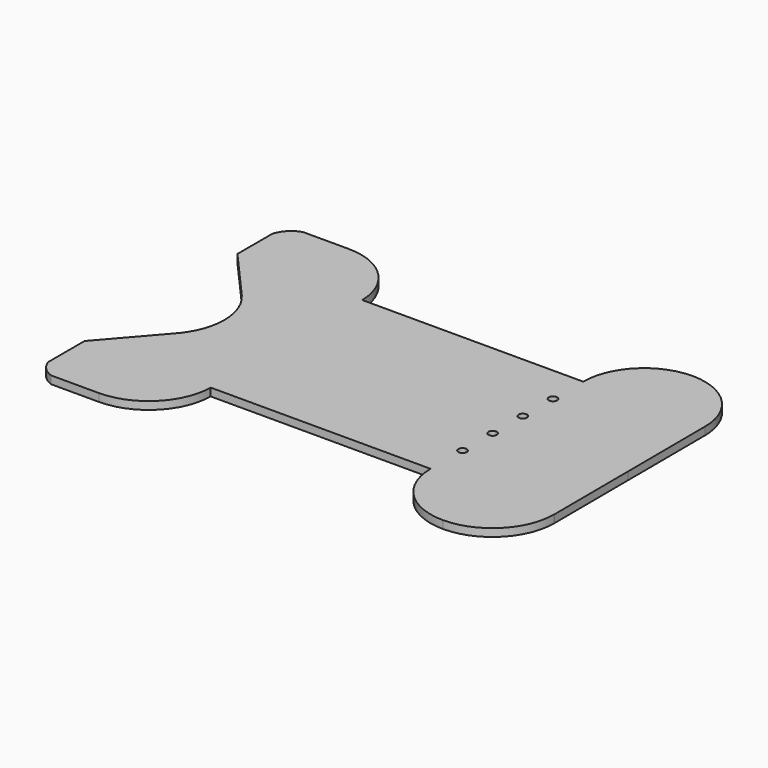
from build123d import *

# Parameters (mm, degrees)
F1_DEPTH = 3.175


# Not quite as in the source:
# - a length typed as a fraction of an inch, garbled in the dataset ("3 / 203.2 mm" for 3/8 in), is restored
# - a feature names something its author has since deleted; it is built from what else it names


with BuildPart() as f1:
    # F0 (on Top) → F1 (new body)
    with BuildSketch(Plane.XY):
        with BuildLine():
            Line((-58.4220365395, 55.6676574051), (-83.8141146934, 55.6676574051))
            Line((-83.8141146934, 55.6676574051), (-83.8141146934, 17.4082663185))
            Line((-83.8141146934, 17.4082663185), (-54.5982423949, 17.2266236973))
            ThreePointArc((-54.5982423949, 17.2266236973), (-52.878445863, 18.9304561303), (-51.1692755304, 17.2159644142))
            ThreePointArc((-51.1692755304, 17.2159644142), (-51.1692838142, 17.2106347468), (-51.1693086658, 17.205305131))
            Line((-51.1693086658, 17.205305131), (-48.1096365395, 17.1862823595))
            Line((-48.1096365395, 17.1862823595), (-48.1096365395, 55.6676574051))
            Line((-48.1096365395, 55.6676574051), (-51.9196365395, 55.6676574051))
            Line((-51.9196365395, 55.6676574051), (-58.4220365395, 55.6676574051))
        make_face()
        with BuildLine():
            Line((-83.8141146934, 80.4333333333), (-83.8141146934, 55.6676574051))
            Line((-83.8141146934, 55.6676574051), (-58.4220365395, 55.6676574051))
            ThreePointArc((-58.4220365395, 55.6676574051), (-66.0792878183, 73.2167300378), (-83.8141146934, 80.4333333333))
        make_face()
        with BuildLine():
            Line((-96.5141146934, 55.6676574051), (-83.8141146934, 55.6676574051))
            Line((-83.8141146934, 55.6676574051), (-83.8141146934, 80.4333333333))
            Line((-83.8141146934, 80.4333333333), (-96.5141146934, 80.4333333333))
            Line((-96.5141146934, 80.4333333333), (-102.2933936502, 80.4333333333))
            ThreePointArc((-102.2933936502, 80.4333333333), (-106.1483818555, 78.2913178986), (-108.7325867358, 74.7176574051))
            Line((-108.7325867358, 74.7176574051), (-102.8641146934, 74.7176574051))
            Line((-102.8641146934, 74.7176574051), (-99.6891146934, 74.7176574051))
            Line((-99.6891146934, 74.7176574051), (-99.6891146934, 55.6676574051))
            Line((-99.6891146934, 55.6676574051), (-96.5141146934, 55.6676574051))
        make_face()
        with BuildLine():
            Line((-83.8141146934, 17.4082663185), (-83.8141146934, 55.6676574051))
            Line((-83.8141146934, 55.6676574051), (-96.5141146934, 55.6676574051))
            Line((-96.5141146934, 55.6676574051), (-99.6891146934, 55.6676574051))
            Line((-99.6891146934, 55.6676574051), (-102.8641146934, 55.6676574051))
            Line((-102.8641146934, 55.6676574051), (-109.2141146934, 55.6676574051))
            Line((-109.2141146934, 55.6676574051), (-90.4137483739, 34.3826312783))
            ThreePointArc((-90.4137483739, 34.3826312783), (-85.6948772916, 26.5569289565), (-84.0509922302, 17.5676574051))
            ThreePointArc((-84.0509922302, 17.5676574051), (-84.0511149543, 17.4886993707), (-84.0514831256, 17.4097420993))
            Line((-84.0514831256, 17.4097420993), (-83.8141146934, 17.4082663185))
        make_face()
        with BuildLine():
            Line((-54.5982423949, 17.2266236973), (-83.8141146934, 17.4082663185))
            Line((-83.8141146934, 17.4082663185), (-83.8141146934, -21.4370436153))
            Line((-83.8141146934, -21.4370436153), (-58.4141146934, -21.4370436153))
            Line((-58.4141146934, -21.4370436153), (-48.1096365395, -21.4370436153))
            Line((-48.1096365395, -21.4370436153), (-48.1096365395, 17.1862823595))
            Line((-48.1096365395, 17.1862823595), (-51.1693086658, 17.205305131))
            ThreePointArc((-51.1693086658, 17.205305131), (-52.8944348135, 15.5014975496), (-54.5982423949, 17.2266236973))
        make_face()
        with BuildLine():
            Line((-83.8141146934, -21.4370436153), (-83.8141146934, 17.4082663185))
            Line((-83.8141146934, 17.4082663185), (-84.0514831256, 17.4097420993))
            ThreePointArc((-84.0514831256, 17.4097420993), (-85.9174728188, 8.0108031049), (-91.1328551507, -0.0279629004))
            Line((-91.1328551507, -0.0279629004), (-91.0666517454, 0))
            Line((-91.0666517454, 0), (-109.6934945268, -21.4370436153))
            Line((-109.6934945268, -21.4370436153), (-103.5974945268, -21.4370436153))
            Line((-103.5974945268, -21.4370436153), (-100.1684945268, -21.4370436153))
            Line((-100.1684945268, -21.4370436153), (-83.8141146934, -21.4370436153))
        make_face()
        with BuildLine():
            Line((-58.4141146934, -21.4370436153), (-83.8141146934, -21.4370436153))
            Line((-83.8141146934, -21.4370436153), (-83.8141146934, -46.5666666667))
            ThreePointArc((-83.8141146934, -46.5666666667), (-65.9485232906, -39.2230246493), (-58.4141146934, -21.4370436153))
        make_face()
        with BuildLine():
            Line((-83.8141146934, -46.5666666667), (-83.8141146934, -21.4370436153))
            Line((-83.8141146934, -21.4370436153), (-100.1684945268, -21.4370436153))
            Line((-100.1684945268, -21.4370436153), (-100.1684945268, -40.4870436153))
            Line((-100.1684945268, -40.4870436153), (-103.5974945268, -40.4870436153))
            Line((-103.5974945268, -40.4870436153), (-109.4795895949, -40.4870436153))
            ThreePointArc((-109.4795895949, -40.4870436153), (-107.0154315461, -44.2413370786), (-103.1736042979, -46.5666666667))
            Line((-103.1736042979, -46.5666666667), (-96.7538046101, -46.5666666667))
            Line((-96.7538046101, -46.5666666667), (-83.8141146934, -46.5666666667))
        make_face()
        with BuildLine():
            ThreePointArc((-51.1692755304, 17.2159644142), (-52.878445863, 18.9304561303), (-54.5982423949, 17.2266236973))
            Line((-54.5982423949, 17.2266236973), (-51.1693086658, 17.205305131))
            ThreePointArc((-51.1693086658, 17.205305131), (-51.1692838142, 17.2106347468), (-51.1692755304, 17.2159644142))
        make_face()
        with BuildLine():
            Line((-51.1693086658, 17.205305131), (-54.5982423949, 17.2266236973))
            ThreePointArc((-54.5982423949, 17.2266236973), (-52.8944348135, 15.5014975496), (-51.1693086658, 17.205305131))
        make_face()
        with BuildLine():
            Line((56.1858853066, 55.6676574051), (56.1858853066, 80.4333333333))
            ThreePointArc((56.1858853066, 80.4333333333), (38.6739079171, 73.1796347946), (31.4202093784, 55.6676574051))
            Line((31.4202093784, 55.6676574051), (56.1858853066, 55.6676574051))
        make_face()
        with BuildLine():
            ThreePointArc((80.9515612348, 55.6676574051), (73.6978626961, 73.1796347946), (56.1858853066, 80.4333333333))
            Line((56.1858853066, 80.4333333333), (56.1858853066, 55.6676574051))
            Line((56.1858853066, 55.6676574051), (80.9515612348, 55.6676574051))
        make_face()
        with BuildLine():
            Line((-102.8641146934, 55.6676574051), (-99.6891146934, 55.6676574051))
            Line((-99.6891146934, 55.6676574051), (-99.6891146934, 74.7176574051))
            Line((-99.6891146934, 74.7176574051), (-102.8641146934, 74.7176574051))
            Line((-102.8641146934, 74.7176574051), (-102.8641146934, 71.6696574051))
            ThreePointArc((-102.8641146934, 71.6696574051), (-101.651780117, 71.1674919815), (-101.1496146934, 69.9551574051))
            ThreePointArc((-101.1496146934, 69.9551574051), (-101.651780117, 68.7428228288), (-102.8641146934, 68.2406574051))
            Line((-102.8641146934, 68.2406574051), (-102.8641146934, 62.1446574051))
            ThreePointArc((-102.8641146934, 62.1446574051), (-101.651780117, 61.6424919815), (-101.1496146934, 60.4301574051))
            ThreePointArc((-101.1496146934, 60.4301574051), (-101.651780117, 59.2178228288), (-102.8641146934, 58.7156574051))
            Line((-102.8641146934, 58.7156574051), (-102.8641146934, 55.6676574051))
        make_face()
        with BuildLine():
            Line((-100.1684945268, -40.4870436153), (-100.1684945268, -21.4370436153))
            Line((-100.1684945268, -21.4370436153), (-103.5974945268, -21.4370436153))
            Line((-103.5974945268, -21.4370436153), (-103.5974945268, -25.4485957723))
            ThreePointArc((-103.5974945268, -25.4485957723), (-102.3851599505, -25.9507611959), (-101.8829945268, -27.1630957723))
            ThreePointArc((-101.8829945268, -27.1630957723), (-102.3851599505, -28.3754303486), (-103.5974945268, -28.8775957723))
            Line((-103.5974945268, -28.8775957723), (-103.5974945268, -32.9818256598))
            ThreePointArc((-103.5974945268, -32.9818256598), (-102.3851599505, -33.4839910834), (-101.8829945268, -34.6963256598))
            ThreePointArc((-101.8829945268, -34.6963256598), (-102.3851599505, -35.9086602361), (-103.5974945268, -36.4108256598))
            Line((-103.5974945268, -36.4108256598), (-103.5974945268, -40.4870436153))
            Line((-103.5974945268, -40.4870436153), (-100.1684945268, -40.4870436153))
        make_face()
        Polygon((-39.2196365395, 55.6676574051), (-48.1096365395, 55.6676574051), (-48.1096365395, 17.1862823595), (-39.2196365395, 17.1310109342), align=None)
        with BuildLine():
            Line((81.1369927167, 16.382722696), (80.9515612348, 55.6676574051))
            ThreePointArc((80.9515612348, 55.6676574051), (73.6978626961, 38.1556800156), (56.1858853066, 30.9019814769))
            Line((56.1858853066, 30.9019814769), (56.1858853066, 26.6474814769))
            ThreePointArc((56.1858853066, 26.6474814769), (57.398219883, 26.1453160533), (57.9003853066, 24.9329814769))
            ThreePointArc((57.9003853066, 24.9329814769), (57.398219883, 23.7206469006), (56.1858853066, 23.2184814769))
            Line((56.1858853066, 23.2184814769), (56.1858853066, 16.5378501727))
            Line((56.1858853066, 16.5378501727), (81.1369927167, 16.382722696))
        make_face()
        with BuildLine():
            ThreePointArc((56.1858853066, 30.9019814769), (73.6978626961, 38.1556800156), (80.9515612348, 55.6676574051))
            Line((80.9515612348, 55.6676574051), (56.1858853066, 55.6676574051))
            Line((56.1858853066, 55.6676574051), (56.1858853066, 30.9019814769))
        make_face()
        with BuildLine():
            Line((31.35631828, 42.1423083088), (31.4202093784, 55.6676574051))
            Line((31.4202093784, 55.6676574051), (24.2803634605, 55.6676574051))
            Line((24.2803634605, 55.6676574051), (20.4703634605, 55.6676574051))
            Line((20.4703634605, 55.6676574051), (20.4703634605, 16.7599027932))
            Line((20.4703634605, 16.7599027932), (23.5155513145, 16.7409700741))
            ThreePointArc((23.5155513145, 16.7409700741), (25.2353478464, 18.4448025071), (26.944518179, 16.730310791))
            ThreePointArc((26.944518179, 16.730310791), (26.9445098952, 16.7249811236), (26.9444850436, 16.7196515078))
            Line((26.9444850436, 16.7196515078), (31.2361005906, 16.6929694259))
            Line((31.2361005906, 16.6929694259), (31.2681297634, 23.4733465661))
            ThreePointArc((31.2681297634, 23.4733465661), (29.5617477636, 25.1959263091), (31.2843275066, 26.9023083088))
            Line((31.2843275066, 26.9023083088), (31.3401205367, 38.7133465661))
            ThreePointArc((31.3401205367, 38.7133465661), (29.633738537, 40.4359263091), (31.35631828, 42.1423083088))
        make_face()
        with BuildLine():
            Line((56.1858853066, 55.6676574051), (31.4202093784, 55.6676574051))
            ThreePointArc((31.4202093784, 55.6676574051), (38.6739079171, 38.1556800156), (56.1858853066, 30.9019814769))
            Line((56.1858853066, 30.9019814769), (56.1858853066, 55.6676574051))
        make_face()
        with BuildLine():
            ThreePointArc((56.1858853066, 30.9019814769), (38.6739079171, 38.1556800156), (31.4202093784, 55.6676574051))
            Line((31.4202093784, 55.6676574051), (31.35631828, 42.1423083088))
            ThreePointArc((31.35631828, 42.1423083088), (32.5634139947, 41.6372952408), (33.0627194083, 40.4278274374))
            ThreePointArc((33.0627194083, 40.4278274374), (32.5576872116, 39.2126328511), (31.3401205367, 38.7133465661))
            Line((31.3401205367, 38.7133465661), (31.2843275066, 26.9023083088))
            ThreePointArc((31.2843275066, 26.9023083088), (32.4914232214, 26.3972952408), (32.990728635, 25.1878274374))
            ThreePointArc((32.990728635, 25.1878274374), (32.4856964383, 23.9726328511), (31.2681297634, 23.4733465661))
            Line((31.2681297634, 23.4733465661), (31.2361005906, 16.6929694259))
            Line((31.2361005906, 16.6929694259), (56.1858853066, 16.5378501727))
            Line((56.1858853066, 16.5378501727), (56.1858853066, 23.2184814769))
            ThreePointArc((56.1858853066, 23.2184814769), (54.4713853066, 24.9329814769), (56.1858853066, 26.6474814769))
            Line((56.1858853066, 26.6474814769), (56.1858853066, 30.9019814769))
        make_face()
        with BuildLine():
            Line((-109.2141146934, 55.6676574051), (-102.8641146934, 55.6676574051))
            Line((-102.8641146934, 55.6676574051), (-102.8641146934, 58.7156574051))
            ThreePointArc((-102.8641146934, 58.7156574051), (-104.5786146934, 60.4301574051), (-102.8641146934, 62.1446574051))
            Line((-102.8641146934, 62.1446574051), (-102.8641146934, 68.2406574051))
            ThreePointArc((-102.8641146934, 68.2406574051), (-104.5786146934, 69.9551574051), (-102.8641146934, 71.6696574051))
            Line((-102.8641146934, 71.6696574051), (-102.8641146934, 74.7176574051))
            Line((-102.8641146934, 74.7176574051), (-108.7325867358, 74.7176574051))
            ThreePointArc((-108.7325867358, 74.7176574051), (-108.9982771043, 74.0351876591), (-109.2141146934, 73.3353516345))
            Line((-109.2141146934, 73.3353516345), (-109.2141146934, 68.0504953692))
            Line((-109.2141146934, 68.0504953692), (-109.2141146934, 55.6676574051))
        make_face()
        Polygon((-48.1096365395, 17.1862823595), (-48.1096365395, -21.4370436153), (-39.2196365395, -21.4370436153), (-39.2196365395, 17.1310109342), align=None)
        with BuildLine():
            Line((-103.5974945268, -25.4485957723), (-103.5974945268, -21.4370436153))
            Line((-103.5974945268, -21.4370436153), (-109.6934945268, -21.4370436153))
            Line((-109.6934945268, -21.4370436153), (-109.6934945268, -34.001855141))
            Line((-109.6934945268, -34.001855141), (-109.6934945268, -39.8522517564))
            ThreePointArc((-109.6934945268, -39.8522517564), (-109.5917750698, -40.1714110456), (-109.4795895949, -40.4870436153))
            Line((-109.4795895949, -40.4870436153), (-103.5974945268, -40.4870436153))
            Line((-103.5974945268, -40.4870436153), (-103.5974945268, -36.4108256598))
            ThreePointArc((-103.5974945268, -36.4108256598), (-105.3119945268, -34.6963256598), (-103.5974945268, -32.9818256598))
            Line((-103.5974945268, -32.9818256598), (-103.5974945268, -28.8775957723))
            ThreePointArc((-103.5974945268, -28.8775957723), (-105.3119945268, -27.1630957723), (-103.5974945268, -25.4485957723))
        make_face()
        with BuildLine():
            Line((11.5803634605, 55.6676574051), (-39.2196365395, 55.6676574051))
            Line((-39.2196365395, 55.6676574051), (-39.2196365395, 17.1310109342))
            Line((-39.2196365395, 17.1310109342), (-36.1589034041, 17.1119815661))
            ThreePointArc((-36.1589034041, 17.1119815661), (-34.4391068722, 18.815813999), (-32.7299365395, 17.1013222829))
            ThreePointArc((-32.7299365395, 17.1013222829), (-32.7299448234, 17.0959926156), (-32.729969675, 17.0906629998))
            Line((-32.729969675, 17.0906629998), (5.0906965959, 16.8555221529))
            ThreePointArc((5.0906965959, 16.8555221529), (6.8104931278, 18.5593545859), (8.5196634605, 16.8448628697))
            ThreePointArc((8.5196634605, 16.8448628697), (8.5196551766, 16.8395332024), (8.519630325, 16.8342035866))
            Line((8.519630325, 16.8342035866), (11.5803634605, 16.8151742185))
            Line((11.5803634605, 16.8151742185), (11.5803634605, 55.6676574051))
        make_face()
        with BuildLine():
            Line((81.3143886077, -21.1998168282), (81.1369927167, 16.382722696))
            Line((81.1369927167, 16.382722696), (56.1858853066, 16.5378501727))
            Line((56.1858853066, 16.5378501727), (56.1858853066, 13.1854814769))
            ThreePointArc((56.1858853066, 13.1854814769), (57.398219883, 12.6833160533), (57.9003853066, 11.4709814769))
            ThreePointArc((57.9003853066, 11.4709814769), (57.398219883, 10.2586469006), (56.1858853066, 9.7564814769))
            Line((56.1858853066, 9.7564814769), (56.1858853066, 3.692579436))
            ThreePointArc((56.1858853066, 3.692579436), (73.8711409588, -3.5840414247), (81.3143886077, -21.1998168282))
        make_face()
        with BuildLine():
            ThreePointArc((-102.8641146934, 62.1446574051), (-104.5786146934, 60.4301574051), (-102.8641146934, 58.7156574051))
            Line((-102.8641146934, 58.7156574051), (-102.8641146934, 62.1446574051))
        make_face()
        with BuildLine():
            Line((-102.8641146934, 62.1446574051), (-102.8641146934, 58.7156574051))
            ThreePointArc((-102.8641146934, 58.7156574051), (-101.651780117, 59.2178228288), (-101.1496146934, 60.4301574051))
            ThreePointArc((-101.1496146934, 60.4301574051), (-101.651780117, 61.6424919815), (-102.8641146934, 62.1446574051))
        make_face()
        with BuildLine():
            Line((-39.2196365395, 17.1310109342), (-39.2196365395, -21.4370436153))
            Line((-39.2196365395, -21.4370436153), (11.5803634605, -21.4370436153))
            Line((11.5803634605, -21.4370436153), (11.5803634605, 16.8151742185))
            Line((11.5803634605, 16.8151742185), (8.519630325, 16.8342035866))
            ThreePointArc((8.519630325, 16.8342035866), (6.7945041773, 15.1303960052), (5.0906965959, 16.8555221529))
            Line((5.0906965959, 16.8555221529), (-32.729969675, 17.0906629998))
            ThreePointArc((-32.729969675, 17.0906629998), (-34.4550958227, 15.3868554184), (-36.1589034041, 17.1119815661))
            Line((-36.1589034041, 17.1119815661), (-39.2196365395, 17.1310109342))
        make_face()
        with BuildLine():
            Line((56.1858853066, -21.4370436153), (56.1858853066, -46.5666666667))
            ThreePointArc((56.1858853066, -46.5666666667), (73.9552121749, -39.2063704836), (81.315508358, -21.4370436153))
            Line((81.315508358, -21.4370436153), (56.1858853066, -21.4370436153))
        make_face()
        with BuildLine():
            ThreePointArc((31.0562622553, -21.4370436153), (38.4165584384, -39.2063704836), (56.1858853066, -46.5666666667))
            Line((56.1858853066, -46.5666666667), (56.1858853066, -21.4370436153))
            Line((56.1858853066, -21.4370436153), (31.0562622553, -21.4370436153))
        make_face()
        with BuildLine():
            ThreePointArc((-101.8829945268, -27.1630957723), (-102.3851599505, -25.9507611959), (-103.5974945268, -25.4485957723))
            Line((-103.5974945268, -25.4485957723), (-103.5974945268, -28.8775957723))
            ThreePointArc((-103.5974945268, -28.8775957723), (-102.3851599505, -28.3754303486), (-101.8829945268, -27.1630957723))
        make_face()
        with BuildLine():
            Line((-103.5974945268, -28.8775957723), (-103.5974945268, -25.4485957723))
            ThreePointArc((-103.5974945268, -25.4485957723), (-105.3119945268, -27.1630957723), (-103.5974945268, -28.8775957723))
        make_face()
        Polygon((20.4703634605, 55.6676574051), (11.5803634605, 55.6676574051), (11.5803634605, 16.8151742185), (20.4703634605, 16.7599027932), align=None)
        with BuildLine():
            ThreePointArc((57.9003853066, 24.9329814769), (57.398219883, 26.1453160533), (56.1858853066, 26.6474814769))
            Line((56.1858853066, 26.6474814769), (56.1858853066, 23.2184814769))
            ThreePointArc((56.1858853066, 23.2184814769), (57.398219883, 23.7206469006), (57.9003853066, 24.9329814769))
        make_face()
        with BuildLine():
            Line((56.1858853066, 23.2184814769), (56.1858853066, 26.6474814769))
            ThreePointArc((56.1858853066, 26.6474814769), (54.4713853066, 24.9329814769), (56.1858853066, 23.2184814769))
        make_face()
        with BuildLine():
            Line((81.315508358, -21.4370436153), (81.3143886077, -21.1998168282))
            ThreePointArc((81.3143886077, -21.1998168282), (73.8711409588, -3.5840414247), (56.1858853066, 3.692579436))
            Line((56.1858853066, 3.692579436), (56.1858853066, -21.4370436153))
            Line((56.1858853066, -21.4370436153), (81.315508358, -21.4370436153))
        make_face()
        with BuildLine():
            ThreePointArc((81.315508358, -21.4370436153), (81.3152284188, -21.3184289004), (81.3143886077, -21.1998168282))
            Line((81.3143886077, -21.1998168282), (81.315508358, -21.4370436153))
        make_face()
        with BuildLine():
            Line((56.1858853066, 13.1854814769), (56.1858853066, 16.5378501727))
            Line((56.1858853066, 16.5378501727), (31.2361005906, 16.6929694259))
            Line((31.2361005906, 16.6929694259), (31.2123367333, 11.6623083088))
            ThreePointArc((31.2123367333, 11.6623083088), (32.4194324481, 11.1572952408), (32.9187378617, 9.9478274374))
            ThreePointArc((32.9187378617, 9.9478274374), (32.413705665, 8.7326328511), (31.1961389901, 8.2333465661))
            Line((31.1961389901, 8.2333465661), (31.14034596, -3.5776916912))
            ThreePointArc((31.14034596, -3.5776916912), (32.3474416748, -4.0827047592), (32.8467470884, -5.2921725626))
            ThreePointArc((32.8467470884, -5.2921725626), (32.3417148917, -6.5073671489), (31.1241482168, -7.0066534339))
            Line((31.1241482168, -7.0066534339), (31.0565426242, -21.3183378707))
            ThreePointArc((31.0565426242, -21.3183378707), (38.4585769367, -3.6257973743), (56.1858853066, 3.692579436))
            Line((56.1858853066, 3.692579436), (56.1858853066, 9.7564814769))
            ThreePointArc((56.1858853066, 9.7564814769), (54.4713853066, 11.4709814769), (56.1858853066, 13.1854814769))
        make_face()
        with BuildLine():
            ThreePointArc((-101.1496146934, 69.9551574051), (-101.651780117, 71.1674919815), (-102.8641146934, 71.6696574051))
            Line((-102.8641146934, 71.6696574051), (-102.8641146934, 68.2406574051))
            ThreePointArc((-102.8641146934, 68.2406574051), (-101.651780117, 68.7428228288), (-101.1496146934, 69.9551574051))
        make_face()
        with BuildLine():
            Line((-102.8641146934, 68.2406574051), (-102.8641146934, 71.6696574051))
            ThreePointArc((-102.8641146934, 71.6696574051), (-104.5786146934, 69.9551574051), (-102.8641146934, 68.2406574051))
        make_face()
        Polygon((11.5803634605, 16.8151742185), (11.5803634605, -21.4370436153), (20.4703634605, -21.4370436153), (20.4703634605, 16.7599027932), align=None)
        with BuildLine():
            ThreePointArc((31.0565426242, -21.3183378707), (31.0563323476, -21.3776905775), (31.0562622553, -21.4370436153))
            Line((31.0562622553, -21.4370436153), (56.1858853066, -21.4370436153))
            Line((56.1858853066, -21.4370436153), (56.1858853066, 3.692579436))
            ThreePointArc((56.1858853066, 3.692579436), (38.4585769367, -3.6257973743), (31.0565426242, -21.3183378707))
        make_face()
        with BuildLine():
            ThreePointArc((-103.5974945268, -32.9818256598), (-105.3119945268, -34.6963256598), (-103.5974945268, -36.4108256598))
            Line((-103.5974945268, -36.4108256598), (-103.5974945268, -32.9818256598))
        make_face()
        with BuildLine():
            Line((-103.5974945268, -32.9818256598), (-103.5974945268, -36.4108256598))
            ThreePointArc((-103.5974945268, -36.4108256598), (-102.3851599505, -35.9086602361), (-101.8829945268, -34.6963256598))
            ThreePointArc((-101.8829945268, -34.6963256598), (-102.3851599505, -33.4839910834), (-103.5974945268, -32.9818256598))
        make_face()
        with BuildLine():
            ThreePointArc((-32.7299365395, 17.1013222829), (-34.4391068722, 18.815813999), (-36.1589034041, 17.1119815661))
            Line((-36.1589034041, 17.1119815661), (-32.729969675, 17.0906629998))
            ThreePointArc((-32.729969675, 17.0906629998), (-32.7299448234, 17.0959926156), (-32.7299365395, 17.1013222829))
        make_face()
        with BuildLine():
            Line((-32.729969675, 17.0906629998), (-36.1589034041, 17.1119815661))
            ThreePointArc((-36.1589034041, 17.1119815661), (-34.4550958227, 15.3868554184), (-32.729969675, 17.0906629998))
        make_face()
        with BuildLine():
            ThreePointArc((57.9003853066, 11.4709814769), (57.398219883, 12.6833160533), (56.1858853066, 13.1854814769))
            Line((56.1858853066, 13.1854814769), (56.1858853066, 9.7564814769))
            ThreePointArc((56.1858853066, 9.7564814769), (57.398219883, 10.2586469006), (57.9003853066, 11.4709814769))
        make_face()
        with BuildLine():
            Line((56.1858853066, 9.7564814769), (56.1858853066, 13.1854814769))
            ThreePointArc((56.1858853066, 13.1854814769), (54.4713853066, 11.4709814769), (56.1858853066, 9.7564814769))
        make_face()
        with BuildLine():
            Line((31.2123367333, 11.6623083088), (31.2361005906, 16.6929694259))
            Line((31.2361005906, 16.6929694259), (26.9444850436, 16.7196515078))
            ThreePointArc((26.9444850436, 16.7196515078), (25.2193588959, 15.0158439264), (23.5155513145, 16.7409700741))
            Line((23.5155513145, 16.7409700741), (20.4703634605, 16.7599027932))
            Line((20.4703634605, 16.7599027932), (20.4703634605, -21.4370436153))
            Line((20.4703634605, -21.4370436153), (31.0559818816, -21.4370436153))
            Line((31.0559818816, -21.4370436153), (31.0565426242, -21.3183378707))
            Line((31.0565426242, -21.3183378707), (31.1241482168, -7.0066534339))
            ThreePointArc((31.1241482168, -7.0066534339), (29.417766217, -5.2840736909), (31.14034596, -3.5776916912))
            Line((31.14034596, -3.5776916912), (31.1961389901, 8.2333465661))
            ThreePointArc((31.1961389901, 8.2333465661), (29.4897569903, 9.9559263091), (31.2123367333, 11.6623083088))
        make_face()
        with BuildLine():
            ThreePointArc((5.0906965959, 16.8555221529), (6.7945041773, 15.1303960052), (8.519630325, 16.8342035866))
            Line((8.519630325, 16.8342035866), (5.0906965959, 16.8555221529))
        make_face()
        with BuildLine():
            Line((5.0906965959, 16.8555221529), (8.519630325, 16.8342035866))
            ThreePointArc((8.519630325, 16.8342035866), (8.5196551766, 16.8395332024), (8.5196634605, 16.8448628697))
            ThreePointArc((8.5196634605, 16.8448628697), (6.8104931278, 18.5593545859), (5.0906965959, 16.8555221529))
        make_face()
        with BuildLine():
            ThreePointArc((23.5155513145, 16.7409700741), (25.2193588959, 15.0158439264), (26.9444850436, 16.7196515078))
            Line((26.9444850436, 16.7196515078), (23.5155513145, 16.7409700741))
        make_face()
        with BuildLine():
            Line((23.5155513145, 16.7409700741), (26.9444850436, 16.7196515078))
            ThreePointArc((26.9444850436, 16.7196515078), (26.9445098952, 16.7249811236), (26.944518179, 16.730310791))
            ThreePointArc((26.944518179, 16.730310791), (25.2353478464, 18.4448025071), (23.5155513145, 16.7409700741))
        make_face()
    extrude(amount=F1_DEPTH)


solid = f1.part
